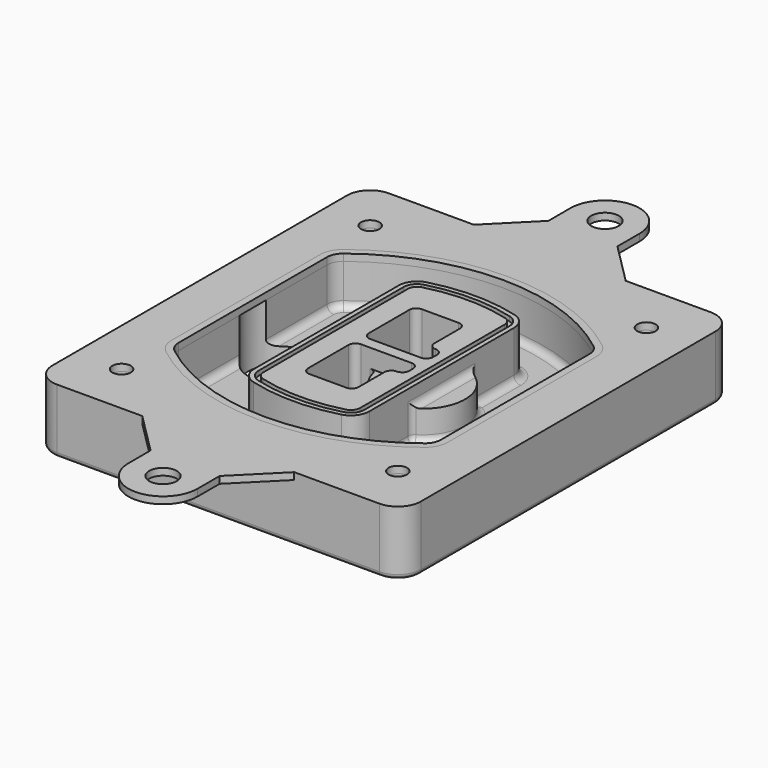
from build123d import *

# Parameters (mm, degrees)
F0_R      = 4
F1_DEPTH  = 25
F2_DEPTH  = 3
F3_DEPTH  = 18
F5_DEPTH  = 21
F6_DEPTH  = 2
F8_DEPTH  = 20
F9_DEPTH  = 16
F10_DEPTH = 25
F7_R      = 6
F7_R_2    = 4
F11_DEPTH = 6
F13_DEPTH = 9
F14_R     = 3
F15_R     = 2
F16_R     = 6
F16_R_2   = 4
F17_DEPTH = 3


with BuildPart() as f1:
    # F0 (on Top) → F1 (new body)
    with BuildSketch(Plane.XY):
        with BuildLine():
            ThreePointArc((-80, -80), (-77.0710678119, -87.0710678119), (-70, -90))
            Line((-70, -90), (70, -90))
            ThreePointArc((70, -90), (77.0710678119, -87.0710678119), (80, -80))
            Line((80, -80), (80, 80))
            ThreePointArc((80, 80), (77.0710678119, 87.0710678119), (70, 90))
            Line((70, 90), (-70, 90))
            ThreePointArc((-70, 90), (-77.0710678119, 87.0710678119), (-80, 80))
            Line((-80, 80), (-80, -80))
        make_face()
        with Locations((-60, -67.5)):
            Circle(F0_R, mode=Mode.SUBTRACT)
        with Locations((60, -67.5)):
            Circle(F0_R, mode=Mode.SUBTRACT)
        with Locations((-60, 67.5)):
            Circle(F0_R, mode=Mode.SUBTRACT)
        with BuildLine():
            ThreePointArc((-64, 40.2934422872), (-62.5820384798, 46.4328484224), (-58.6153846154, 51.3286200352))
            ThreePointArc((-58.6153846154, 51.3286200352), (0, 71.5), (58.6153846154, 51.3286200352))
            ThreePointArc((58.6153846154, 51.3286200352), (62.5820384798, 46.4328484224), (64, 40.2934422872))
            Line((64, 40.2934422872), (64, -40.2934422872))
            ThreePointArc((64, -40.2934422872), (62.5820384798, -46.4328484224), (58.6153846154, -51.3286200352))
            ThreePointArc((58.6153846154, -51.3286200352), (0, -71.5), (-58.6153846154, -51.3286200352))
            ThreePointArc((-58.6153846154, -51.3286200352), (-62.5820384798, -46.4328484224), (-64, -40.2934422872))
            Line((-64, -40.2934422872), (-64, 40.2934422872))
        make_face(mode=Mode.SUBTRACT)
        with Locations((60, 67.5)):
            Circle(F0_R, mode=Mode.SUBTRACT)
        with BuildLine():
            ThreePointArc((58.6153846154, 51.3286200352), (0, 71.5), (-58.6153846154, 51.3286200352))
            ThreePointArc((-58.6153846154, 51.3286200352), (-62.5820384798, 46.4328484224), (-64, 40.2934422872))
            Line((-64, 40.2934422872), (-64, -40.2934422872))
            ThreePointArc((-64, -40.2934422872), (-62.5820384798, -46.4328484224), (-58.6153846154, -51.3286200352))
            ThreePointArc((-58.6153846154, -51.3286200352), (0, -71.5), (58.6153846154, -51.3286200352))
            ThreePointArc((58.6153846154, -51.3286200352), (62.5820384798, -46.4328484224), (64, -40.2934422872))
            Line((64, -40.2934422872), (64, 40.2934422872))
            ThreePointArc((64, 40.2934422872), (62.5820384798, 46.4328484224), (58.6153846154, 51.3286200352))
        make_face()
        with BuildLine():
            Line((-60, -40.2934422872), (-60, 40.2934422872))
            ThreePointArc((-60, 40.2934422872), (-58.9871703427, 44.6787323838), (-56.1538461538, 48.1757121072))
            ThreePointArc((-56.1538461538, 48.1757121072), (0, 67.5), (56.1538461538, 48.1757121072))
            ThreePointArc((56.1538461538, 48.1757121072), (58.9871703427, 44.6787323838), (60, 40.2934422872))
            Line((60, 40.2934422872), (60, -40.2934422872))
            ThreePointArc((60, -40.2934422872), (58.9871703427, -44.6787323838), (56.1538461538, -48.1757121072))
            ThreePointArc((56.1538461538, -48.1757121072), (0, -67.5), (-56.1538461538, -48.1757121072))
            ThreePointArc((-56.1538461538, -48.1757121072), (-58.9871703427, -44.6787323838), (-60, -40.2934422872))
        make_face(mode=Mode.SUBTRACT)
        with BuildLine():
            ThreePointArc((-56.1538461538, 48.1757121072), (-58.9871703427, 44.6787323838), (-60, 40.2934422872))
            Line((-60, 40.2934422872), (-60, -40.2934422872))
            ThreePointArc((-60, -40.2934422872), (-58.9871703427, -44.6787323838), (-56.1538461538, -48.1757121072))
            ThreePointArc((-56.1538461538, -48.1757121072), (0, -67.5), (56.1538461538, -48.1757121072))
            ThreePointArc((56.1538461538, -48.1757121072), (58.9871703427, -44.6787323838), (60, -40.2934422872))
            Line((60, -40.2934422872), (60, 40.2934422872))
            ThreePointArc((60, 40.2934422872), (58.9871703427, 44.6787323838), (56.1538461538, 48.1757121072))
            ThreePointArc((56.1538461538, 48.1757121072), (0, 67.5), (-56.1538461538, 48.1757121072))
        make_face()
        with BuildLine():
            ThreePointArc((54.3076923077, 45.8110311612), (56.2910192399, 43.3631453548), (57, 40.2934422872))
            Line((57, 40.2934422872), (57, -40.2934422872))
            ThreePointArc((57, -40.2934422872), (56.2910192399, -43.3631453548), (54.3076923077, -45.8110311612))
            ThreePointArc((54.3076923077, -45.8110311612), (0, -64.5), (-54.3076923077, -45.8110311612))
            ThreePointArc((-54.3076923077, -45.8110311612), (-56.2910192399, -43.3631453548), (-57, -40.2934422872))
            Line((-57, -40.2934422872), (-57, 40.2934422872))
            ThreePointArc((-57, 40.2934422872), (-56.2910192399, 43.3631453548), (-54.3076923077, 45.8110311612))
            ThreePointArc((-54.3076923077, 45.8110311612), (0, 64.5), (54.3076923077, 45.8110311612))
        make_face(mode=Mode.SUBTRACT)
        with BuildLine():
            Line((57, -40.2934422872), (57, 40.2934422872))
            ThreePointArc((57, 40.2934422872), (56.2910192399, 43.3631453548), (54.3076923077, 45.8110311612))
            ThreePointArc((54.3076923077, 45.8110311612), (0, 64.5), (-54.3076923077, 45.8110311612))
            ThreePointArc((-54.3076923077, 45.8110311612), (-56.2910192399, 43.3631453548), (-57, 40.2934422872))
            Line((-57, 40.2934422872), (-57, -40.2934422872))
            ThreePointArc((-57, -40.2934422872), (-56.2910192399, -43.3631453548), (-54.3076923077, -45.8110311612))
            ThreePointArc((-54.3076923077, -45.8110311612), (0, -64.5), (54.3076923077, -45.8110311612))
            ThreePointArc((54.3076923077, -45.8110311612), (56.2910192399, -43.3631453548), (57, -40.2934422872))
        make_face()
    extrude(amount=-F1_DEPTH)

    # F0 (on Top) → F3 (cut)
    with BuildSketch(Plane.XY):
        with BuildLine():
            Line((57, -40.2934422872), (57, 40.2934422872))
            ThreePointArc((57, 40.2934422872), (56.2910192399, 43.3631453548), (54.3076923077, 45.8110311612))
            ThreePointArc((54.3076923077, 45.8110311612), (0, 64.5), (-54.3076923077, 45.8110311612))
            ThreePointArc((-54.3076923077, 45.8110311612), (-56.2910192399, 43.3631453548), (-57, 40.2934422872))
            Line((-57, 40.2934422872), (-57, -40.2934422872))
            ThreePointArc((-57, -40.2934422872), (-56.2910192399, -43.3631453548), (-54.3076923077, -45.8110311612))
            ThreePointArc((-54.3076923077, -45.8110311612), (0, -64.5), (54.3076923077, -45.8110311612))
            ThreePointArc((54.3076923077, -45.8110311612), (56.2910192399, -43.3631453548), (57, -40.2934422872))
        make_face()
    extrude(amount=-F3_DEPTH, mode=Mode.SUBTRACT)

    # F4 (on face) → F5 (join, through all)
    with BuildSketch(Plane.XY.offset(3)):
        with BuildLine():
            ThreePointArc((-25, -39.2465276821), (-23.3511545998, -44.1109737193), (-19.0842911877, -46.9702398883))
            ThreePointArc((-19.0842911877, -46.9702398883), (0, -49.5), (19.0842911877, -46.9702398883))
            ThreePointArc((19.0842911877, -46.9702398883), (23.3511545998, -44.1109737193), (25, -39.2465276821))
            Line((25, -39.2465276821), (25, 39.2465276821))
            ThreePointArc((25, 39.2465276821), (23.3511545998, 44.1109737193), (19.0842911877, 46.9702398883))
            ThreePointArc((19.0842911877, 46.9702398883), (0, 49.5), (-19.0842911877, 46.9702398883))
            ThreePointArc((-19.0842911877, 46.9702398883), (-23.3511545998, 44.1109737193), (-25, 39.2465276821))
            Line((-25, 39.2465276821), (-25, -39.2465276821))
        make_face()
        with BuildLine():
            ThreePointArc((18.5632183908, 45.0393118368), (21.7633659499, 42.89486221), (23, 39.2465276821))
            Line((23, 39.2465276821), (23, -39.2465276821))
            ThreePointArc((23, -39.2465276821), (21.7633659499, -42.89486221), (18.5632183908, -45.0393118368))
            ThreePointArc((18.5632183908, -45.0393118368), (0, -47.5), (-18.5632183908, -45.0393118368))
            ThreePointArc((-18.5632183908, -45.0393118368), (-21.7633659499, -42.89486221), (-23, -39.2465276821))
            Line((-23, -39.2465276821), (-23, 39.2465276821))
            ThreePointArc((-23, 39.2465276821), (-21.7633659499, 42.89486221), (-18.5632183908, 45.0393118368))
            ThreePointArc((-18.5632183908, 45.0393118368), (0, 47.5), (18.5632183908, 45.0393118368))
        make_face(mode=Mode.SUBTRACT)
        with BuildLine():
            Line((23, -39.2465276821), (23, 39.2465276821))
            ThreePointArc((23, 39.2465276821), (21.7633659499, 42.89486221), (18.5632183908, 45.0393118368))
            ThreePointArc((18.5632183908, 45.0393118368), (0, 47.5), (-18.5632183908, 45.0393118368))
            ThreePointArc((-18.5632183908, 45.0393118368), (-21.7633659499, 42.89486221), (-23, 39.2465276821))
            Line((-23, 39.2465276821), (-23, -39.2465276821))
            ThreePointArc((-23, -39.2465276821), (-21.7633659499, -42.89486221), (-18.5632183908, -45.0393118368))
            ThreePointArc((-18.5632183908, -45.0393118368), (0, -47.5), (18.5632183908, -45.0393118368))
            ThreePointArc((18.5632183908, -45.0393118368), (21.7633659499, -42.89486221), (23, -39.2465276821))
        make_face()
        with BuildLine():
            ThreePointArc((18.0421455939, 43.1083837852), (20.1755772999, 41.6787507007), (21, 39.2465276821))
            Line((21, 39.2465276821), (21, -39.2465276821))
            ThreePointArc((21, -39.2465276821), (20.1755772999, -41.6787507007), (18.0421455939, -43.1083837852))
            ThreePointArc((18.0421455939, -43.1083837852), (0, -45.5), (-18.0421455939, -43.1083837852))
            ThreePointArc((-18.0421455939, -43.1083837852), (-20.1755772999, -41.6787507007), (-21, -39.2465276821))
            Line((-21, -39.2465276821), (-21, 39.2465276821))
            ThreePointArc((-21, 39.2465276821), (-20.1755772999, 41.6787507007), (-18.0421455939, 43.1083837852))
            ThreePointArc((-18.0421455939, 43.1083837852), (0, 45.5), (18.0421455939, 43.1083837852))
        make_face(mode=Mode.SUBTRACT)
        with BuildLine():
            Line((21, -39.2465276821), (21, 39.2465276821))
            ThreePointArc((21, 39.2465276821), (20.1755772999, 41.6787507007), (18.0421455939, 43.1083837852))
            ThreePointArc((18.0421455939, 43.1083837852), (0, 45.5), (-18.0421455939, 43.1083837852))
            ThreePointArc((-18.0421455939, 43.1083837852), (-20.1755772999, 41.6787507007), (-21, 39.2465276821))
            Line((-21, 39.2465276821), (-21, -39.2465276821))
            ThreePointArc((-21, -39.2465276821), (-20.1755772999, -41.6787507007), (-18.0421455939, -43.1083837852))
            ThreePointArc((-18.0421455939, -43.1083837852), (0, -45.5), (18.0421455939, -43.1083837852))
            ThreePointArc((18.0421455939, -43.1083837852), (20.1755772999, -41.6787507007), (21, -39.2465276821))
        make_face()
        with BuildLine():
            Line((-8, -2.5), (14, -2.5))
            ThreePointArc((14, -2.5), (16.1213203436, -3.3786796564), (17, -5.5))
            Line((17, -5.5), (17, -7.5))
            ThreePointArc((17, -7.5), (16.1213203436, -9.6213203436), (14, -10.5))
            ThreePointArc((14, -10.5), (11.8786796564, -11.3786796564), (11, -13.5))
            Line((11, -13.5), (11, -27.5))
            ThreePointArc((11, -27.5), (10.1213203436, -29.6213203436), (8, -30.5))
            Line((8, -30.5), (-8, -30.5))
            ThreePointArc((-8, -30.5), (-10.1213203436, -29.6213203436), (-11, -27.5))
            Line((-11, -27.5), (-11, -5.5))
            ThreePointArc((-11, -5.5), (-10.1213203436, -3.3786796564), (-8, -2.5))
        make_face(mode=Mode.SUBTRACT)
        with BuildLine():
            ThreePointArc((-8, 2.5), (-10.1213203436, 3.3786796564), (-11, 5.5))
            Line((-11, 5.5), (-11, 27.5))
            ThreePointArc((-11, 27.5), (-10.1213203436, 29.6213203436), (-8, 30.5))
            Line((-8, 30.5), (8, 30.5))
            ThreePointArc((8, 30.5), (10.1213203436, 29.6213203436), (11, 27.5))
            Line((11, 27.5), (11, 13.5))
            ThreePointArc((11, 13.5), (11.8786796564, 11.3786796564), (14, 10.5))
            ThreePointArc((14, 10.5), (16.1213203436, 9.6213203436), (17, 7.5))
            Line((17, 7.5), (17, 5.5))
            ThreePointArc((17, 5.5), (16.1213203436, 3.3786796564), (14, 2.5))
            Line((14, 2.5), (-8, 2.5))
        make_face(mode=Mode.SUBTRACT)
    extrude(amount=-F5_DEPTH)

    # F4 (on face) → F6 (cut)
    with BuildSketch(Plane.XY.offset(3)):
        with BuildLine():
            Line((23, -39.2465276821), (23, 39.2465276821))
            ThreePointArc((23, 39.2465276821), (21.7633659499, 42.89486221), (18.5632183908, 45.0393118368))
            ThreePointArc((18.5632183908, 45.0393118368), (0, 47.5), (-18.5632183908, 45.0393118368))
            ThreePointArc((-18.5632183908, 45.0393118368), (-21.7633659499, 42.89486221), (-23, 39.2465276821))
            Line((-23, 39.2465276821), (-23, -39.2465276821))
            ThreePointArc((-23, -39.2465276821), (-21.7633659499, -42.89486221), (-18.5632183908, -45.0393118368))
            ThreePointArc((-18.5632183908, -45.0393118368), (0, -47.5), (18.5632183908, -45.0393118368))
            ThreePointArc((18.5632183908, -45.0393118368), (21.7633659499, -42.89486221), (23, -39.2465276821))
        make_face()
        with BuildLine():
            ThreePointArc((18.0421455939, 43.1083837852), (20.1755772999, 41.6787507007), (21, 39.2465276821))
            Line((21, 39.2465276821), (21, -39.2465276821))
            ThreePointArc((21, -39.2465276821), (20.1755772999, -41.6787507007), (18.0421455939, -43.1083837852))
            ThreePointArc((18.0421455939, -43.1083837852), (0, -45.5), (-18.0421455939, -43.1083837852))
            ThreePointArc((-18.0421455939, -43.1083837852), (-20.1755772999, -41.6787507007), (-21, -39.2465276821))
            Line((-21, -39.2465276821), (-21, 39.2465276821))
            ThreePointArc((-21, 39.2465276821), (-20.1755772999, 41.6787507007), (-18.0421455939, 43.1083837852))
            ThreePointArc((-18.0421455939, 43.1083837852), (0, 45.5), (18.0421455939, 43.1083837852))
        make_face(mode=Mode.SUBTRACT)
    extrude(amount=-F6_DEPTH, mode=Mode.SUBTRACT)

    # F7 (on face) → F8 (join)
    with BuildSketch(Plane(origin=(0, 0, -25), x_dir=(1, 0, 0), z_dir=(0, 0, -1))):
        with BuildLine():
            ThreePointArc((3.28842436, 0), (16.7567035675, 13.4682792075), (30.224982775, 0))
            Line((30.224982775, 0), (35.224982775, 0))
            ThreePointArc((35.224982775, 0), (16.7567035675, 18.4682792075), (-1.71157564, 0))
            Line((-1.71157564, 0), (3.28842436, 0))
        make_face()
        with BuildLine():
            Line((3.28842436, 0), (30.224982775, 0))
            ThreePointArc((30.224982775, 0), (16.7567035675, 13.4682792075), (3.28842436, 0))
        make_face()
        with BuildLine():
            ThreePointArc((3.28842436, 0), (16.7567035675, -13.4682792075), (30.224982775, 0))
            Line((30.224982775, 0), (3.28842436, 0))
        make_face()
        with BuildLine():
            Line((35.224982775, 0), (30.224982775, 0))
            ThreePointArc((30.224982775, 0), (16.7567035675, -13.4682792075), (3.28842436, 0))
            Line((3.28842436, 0), (-1.71157564, 0))
            ThreePointArc((-1.71157564, 0), (16.7567035675, -18.4682792075), (35.224982775, 0))
        make_face()
    extrude(amount=-F8_DEPTH)

    # F7 (on face) → F9 (cut)
    with BuildSketch(Plane(origin=(0, 0, -25), x_dir=(1, 0, 0), z_dir=(0, 0, -1))):
        with BuildLine():
            Line((3.28842436, 0), (30.224982775, 0))
            ThreePointArc((30.224982775, 0), (16.7567035675, 13.4682792075), (3.28842436, 0))
        make_face()
        with BuildLine():
            ThreePointArc((3.28842436, 0), (16.7567035675, -13.4682792075), (30.224982775, 0))
            Line((30.224982775, 0), (3.28842436, 0))
        make_face()
    extrude(amount=-F9_DEPTH, mode=Mode.SUBTRACT)

    # F7 (on face) → F10 (cut)
    with BuildSketch(Plane(origin=(0, 0, -25), x_dir=(1, 0, 0), z_dir=(0, 0, -1))):
        with BuildLine():
            Line((-59.0318229325, 0), (-32.0952645175, 0))
            ThreePointArc((-32.0952645175, 0), (-45.563543725, 13.4682792075), (-59.0318229325, 0))
        make_face()
        with BuildLine():
            ThreePointArc((-59.0318229325, 0), (-45.563543725, -13.4682792075), (-32.0952645175, 0))
            Line((-32.0952645175, 0), (-59.0318229325, 0))
        make_face()
    extrude(amount=-F10_DEPTH, mode=Mode.SUBTRACT)

    # F7 (on face) → F11 (cut)
    with BuildSketch(Plane(origin=(0, 0, -25), x_dir=(1, 0, 0), z_dir=(0, 0, -1))):
        with Locations((60, -67.5)):
            Circle(F7_R)
        with Locations((60, -67.5)):
            Circle(F7_R_2, mode=Mode.SUBTRACT)
        with Locations((-60, -67.5)):
            Circle(F7_R)
        with Locations((-60, -67.5)):
            Circle(F7_R_2, mode=Mode.SUBTRACT)
        with Locations((-60, 67.5)):
            Circle(F7_R)
        with Locations((-60, 67.5)):
            Circle(F7_R_2, mode=Mode.SUBTRACT)
        with Locations((60, 67.5)):
            Circle(F7_R)
        with Locations((60, 67.5)):
            Circle(F7_R_2, mode=Mode.SUBTRACT)
    extrude(amount=-F11_DEPTH, mode=Mode.SUBTRACT)

    # F12 (on face) → F13 (cut, through all)
    with BuildSketch(Plane(origin=(0, 0, -9), x_dir=(1, 0, 0), z_dir=(0, 0, -1))):
        with BuildLine():
            Line((11, 13.5), (11, 17.5481537753))
            ThreePointArc((11, 17.5481537753), (2.5696536419, 11.8239143813), (-1.5415842455, 2.5))
            Line((-1.5415842455, 2.5), (3.5224848595, 2.5))
            ThreePointArc((3.5224848595, 2.5), (6.1857188154, 8.3455872281), (11.2536447004, 12.2927168648))
            ThreePointArc((11.2536447004, 12.2927168648), (11.0640958889, 12.8831798879), (11, 13.5))
        make_face()
        with BuildLine():
            ThreePointArc((11.2536447004, -12.2927168648), (6.1857188154, -8.3455872281), (3.5224848595, -2.5))
            Line((3.5224848595, -2.5), (-1.5415842455, -2.5))
            ThreePointArc((-1.5415842455, -2.5), (2.5696536419, -11.8239143813), (11, -17.5481537753))
            Line((11, -17.5481537753), (11, -13.5))
            ThreePointArc((11, -13.5), (11.0640958889, -12.8831798879), (11.2536447004, -12.2927168648))
        make_face()
        with BuildLine():
            ThreePointArc((11.2536447004, 12.2927168648), (6.1857188154, 8.3455872281), (3.5224848595, 2.5))
            Line((3.5224848595, 2.5), (14, 2.5))
            ThreePointArc((14, 2.5), (16.1213203436, 3.3786796564), (17, 5.5))
            Line((17, 5.5), (17, 7.5))
            ThreePointArc((17, 7.5), (16.1213203436, 9.6213203436), (14, 10.5))
            ThreePointArc((14, 10.5), (12.3601599782, 10.9878446101), (11.2536447004, 12.2927168648))
        make_face()
        with BuildLine():
            Line((14, -2.5), (3.5224848595, -2.5))
            ThreePointArc((3.5224848595, -2.5), (6.1857188154, -8.3455872281), (11.2536447004, -12.2927168648))
            ThreePointArc((11.2536447004, -12.2927168648), (12.3601599782, -10.9878446101), (14, -10.5))
            ThreePointArc((14, -10.5), (16.1213203436, -9.6213203436), (17, -7.5))
            Line((17, -7.5), (17, -5.5))
            ThreePointArc((17, -5.5), (16.1213203436, -3.3786796564), (14, -2.5))
        make_face()
    extrude(amount=F13_DEPTH, mode=Mode.SUBTRACT)

    # F14
    f14_edges = [f1.edges().sort_by_distance(p)[0] for p in [
        (-57, 23.703476, -18),
        (-57, -23.703476, -18),
        (25, 0, -5),
        (25, 16.526506, -11.5),
        (25, -16.526506, -11.5),
        (25, -27.886517, -18),
        (35.224983, 0, -18),
        (-1.541584, -2.5, -7),
        (-1.541584, 2.5, -7),
        (11, 17.548154, -7),
        (11, -17.548154, -7),
        (23.351155, -44.110974, -18),
        (0, -64.5, -18),
        (-56.291019, -43.363145, -18),
        (-56.291019, 43.363145, -18),
        (0, 64.5, -18),
        (56.291019, 43.363145, -18),
        (57, 0, -18),
        (56.291019, -43.363145, -18),
        (-23.351155, 44.110974, -18),
        (0, 49.5, -18),
        (-25, 0, -18),
        (23.351155, 44.110974, -18),
        (-23.351155, -44.110974, -18),
        (25, 27.886517, -18),
        (0, -49.5, -18),
    ]]
    fillet(f14_edges, radius=F14_R)

    # F15
    f15_edges = [f1.edges().sort_by_distance(p)[0] for p in [
        (0, -90, -25),
        (-77.071068, -87.071068, -25),
        (-80, 0, -25),
        (-77.071068, 87.071068, -25),
        (77.071068, -87.071068, -25),
        (0, 90, -25),
        (80, 0, -25),
        (77.071068, 87.071068, -25),
    ]]
    fillet(f15_edges, radius=F15_R)

    # F16 (on face) → F17 (join, through all)
    with BuildSketch(Plane.XY):
        with BuildLine():
            Line((33, -90), (-33, -90))
            Line((-33, -90), (-15, -108))
            Line((-15, -108), (-15, -120))
            ThreePointArc((-15, -120), (0, -135), (15, -120))
            Line((15, -120), (15, -108))
            Line((15, -108), (33, -90))
        make_face()
        with Locations((0, -120)):
            Circle(F16_R, mode=Mode.SUBTRACT)
        with BuildLine():
            Line((-15, 108), (-33, 90))
            Line((-33, 90), (33, 90))
            Line((33, 90), (15, 108))
            Line((15, 108), (15, 120))
            ThreePointArc((15, 120), (0, 135), (-15, 120))
            Line((-15, 120), (-15, 108))
        make_face()
        with Locations((0, 120)):
            Circle(F16_R, mode=Mode.SUBTRACT)
        with BuildLine():
            Line((33, 90), (-33, 90))
            Line((-33, 90), (-70, 90))
            ThreePointArc((-70, 90), (-77.0710678119, 87.0710678119), (-80, 80))
            Line((-80, 80), (-80, -80))
            ThreePointArc((-80, -80), (-77.0710678119, -87.0710678119), (-70, -90))
            Line((-70, -90), (-33, -90))
            Line((-33, -90), (33, -90))
            Line((33, -90), (70, -90))
            ThreePointArc((70, -90), (77.0710678119, -87.0710678119), (80, -80))
            Line((80, -80), (80, 80))
            ThreePointArc((80, 80), (77.0710678119, 87.0710678119), (70, 90))
            Line((70, 90), (33, 90))
        make_face()
        with Locations((-60, -67.5)):
            Circle(F16_R_2, mode=Mode.SUBTRACT)
        with BuildLine():
            Line((57, 40.2934422872), (57, -40.2934422872))
            ThreePointArc((57, -40.2934422872), (56.2910192399, -43.3631453548), (54.3076923077, -45.8110311612))
            ThreePointArc((54.3076923077, -45.8110311612), (0, -64.5), (-54.3076923077, -45.8110311612))
            ThreePointArc((-54.3076923077, -45.8110311612), (-56.2910192399, -43.3631453548), (-57, -40.2934422872))
            Line((-57, -40.2934422872), (-57, -7.1135091679))
            ThreePointArc((-57, -7.1135091679), (-58.5139091845, -3.6989970638), (-59.0318229325, 0))
            ThreePointArc((-59.0318229325, 0), (-58.5139091845, 3.6989970638), (-57, 7.1135091679))
            Line((-57, 7.1135091679), (-57, 40.2934422872))
            ThreePointArc((-57, 40.2934422872), (-56.2910192399, 43.3631453548), (-54.3076923077, 45.8110311612))
            ThreePointArc((-54.3076923077, 45.8110311612), (0, 64.5), (54.3076923077, 45.8110311612))
            ThreePointArc((54.3076923077, 45.8110311612), (56.2910192399, 43.3631453548), (57, 40.2934422872))
        make_face(mode=Mode.SUBTRACT)
        with Locations((60, -67.5)):
            Circle(F16_R_2, mode=Mode.SUBTRACT)
        with Locations((-60, 67.5)):
            Circle(F16_R_2, mode=Mode.SUBTRACT)
        with Locations((60, 67.5)):
            Circle(F16_R_2, mode=Mode.SUBTRACT)
    extrude(amount=F17_DEPTH)


with BuildPart() as f2:
    # F0 (on Top) → F2 (new body)
    with BuildSketch(Plane.XY):
        with BuildLine():
            ThreePointArc((-56.1538461538, 48.1757121072), (-58.9871703427, 44.6787323838), (-60, 40.2934422872))
            Line((-60, 40.2934422872), (-60, -40.2934422872))
            ThreePointArc((-60, -40.2934422872), (-58.9871703427, -44.6787323838), (-56.1538461538, -48.1757121072))
            ThreePointArc((-56.1538461538, -48.1757121072), (0, -67.5), (56.1538461538, -48.1757121072))
            ThreePointArc((56.1538461538, -48.1757121072), (58.9871703427, -44.6787323838), (60, -40.2934422872))
            Line((60, -40.2934422872), (60, 40.2934422872))
            ThreePointArc((60, 40.2934422872), (58.9871703427, 44.6787323838), (56.1538461538, 48.1757121072))
            ThreePointArc((56.1538461538, 48.1757121072), (0, 67.5), (-56.1538461538, 48.1757121072))
        make_face()
        with BuildLine():
            ThreePointArc((54.3076923077, 45.8110311612), (56.2910192399, 43.3631453548), (57, 40.2934422872))
            Line((57, 40.2934422872), (57, -40.2934422872))
            ThreePointArc((57, -40.2934422872), (56.2910192399, -43.3631453548), (54.3076923077, -45.8110311612))
            ThreePointArc((54.3076923077, -45.8110311612), (0, -64.5), (-54.3076923077, -45.8110311612))
            ThreePointArc((-54.3076923077, -45.8110311612), (-56.2910192399, -43.3631453548), (-57, -40.2934422872))
            Line((-57, -40.2934422872), (-57, 40.2934422872))
            ThreePointArc((-57, 40.2934422872), (-56.2910192399, 43.3631453548), (-54.3076923077, 45.8110311612))
            ThreePointArc((-54.3076923077, 45.8110311612), (0, 64.5), (54.3076923077, 45.8110311612))
        make_face(mode=Mode.SUBTRACT)
    extrude(amount=F2_DEPTH)


solid = Compound([f1.part, f2.part])
